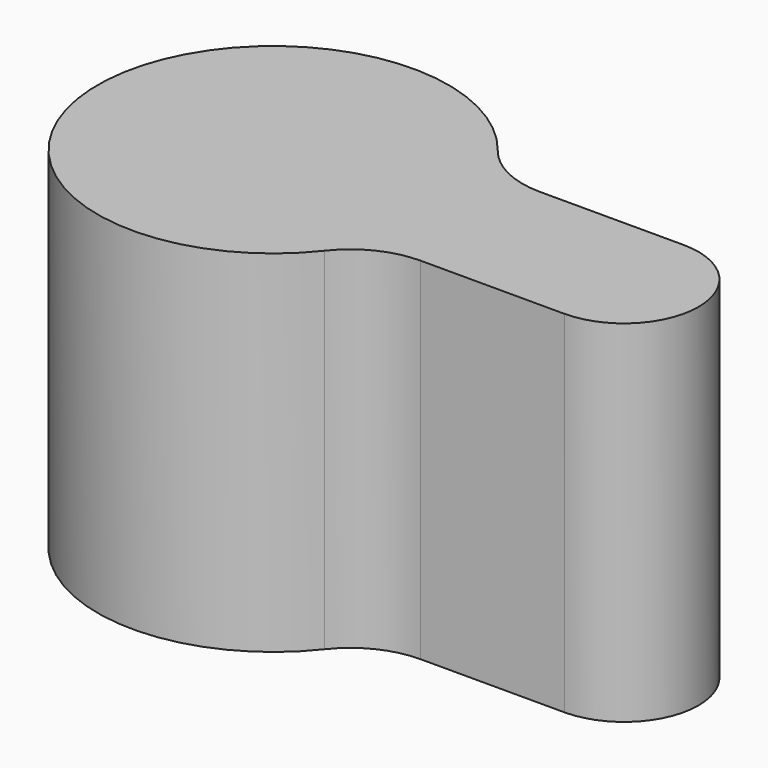
from build123d import *

# Parameters (mm, degrees)
F2_DEPTH = 200


# Not quite as in the source:
# - a feature of the source that left no trace in its solid (it failed there, or was rolled back) is left out


with BuildPart() as f2:
    # F1 (on face) → F2 (new body)
    with BuildSketch(Plane.XY):
        with BuildLine():
            Line((200, 42.5), (118.0836567862, 42.5))
            ThreePointArc((118.0836567862, 42.5), (96.1937808919, 47.5463201358), (78.7224378575, 61.6666666667))
            ThreePointArc((78.7224378575, 61.6666666667), (-100, 0), (78.7224378575, -61.6666666667))
            ThreePointArc((78.7224378575, -61.6666666667), (96.1937808919, -47.5463201358), (118.0836567862, -42.5))
            Line((118.0836567862, -42.5), (200, -42.5))
            ThreePointArc((200, -42.5), (242.5, 0), (200, 42.5))
        make_face()
    extrude(amount=F2_DEPTH)


with BuildPart() as f2b:
    # F0 (on Top) → F2, piece 2 (new body)
    with BuildSketch(Plane.XY):
        with BuildLine():
            ThreePointArc((118.0836567862, 42.5), (96.1937808919, 47.5463201358), (78.7224378575, 61.6666666667))
            ThreePointArc((78.7224378575, 61.6666666667), (-100, 0), (78.7224378575, -61.6666666667))
            ThreePointArc((78.7224378575, -61.6666666667), (96.1937808919, -47.5463201358), (118.0836567862, -42.5))
            Line((118.0836567862, -42.5), (200, -42.5))
            ThreePointArc((200, -42.5), (242.5, 0), (200, 42.5))
            Line((200, 42.5), (118.0836567862, 42.5))
        make_face()
    extrude(amount=F2_DEPTH)


solid = Compound([f2.part, f2b.part])
